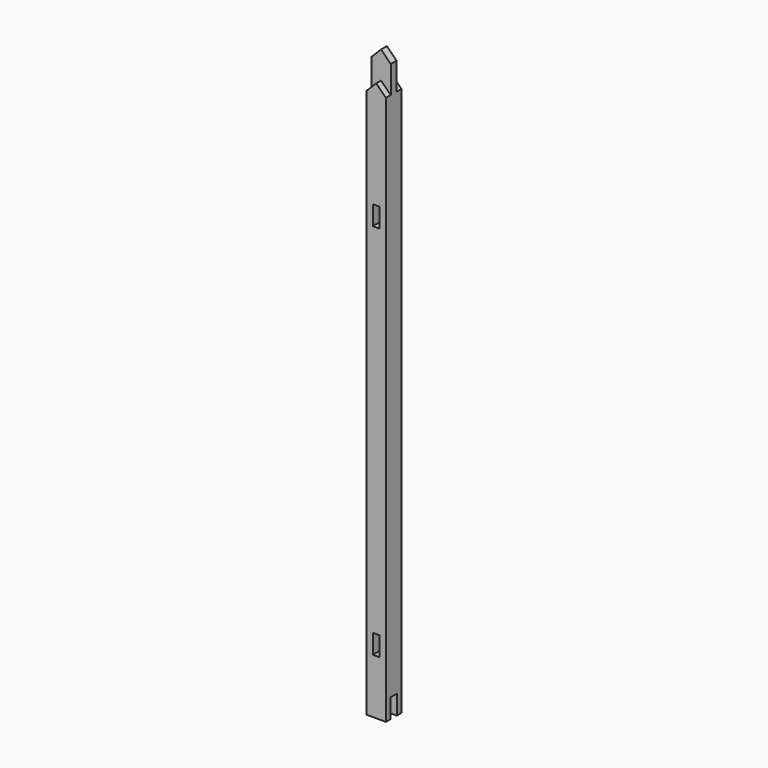
from build123d import *

# Parameters (mm, degrees)
F0_W      = 45
F0_H      = 45
F1_DEPTH  = 650
F3_DEPTH  = 14
F4_W      = 16
F4_H      = 45
F5_DEPTH  = 45.001
F6_W      = 18
F6_H      = 45
F7_DEPTH  = 45.001
F8_W      = 16
F8_H      = 45
F9_DEPTH  = 45.001
F10_W     = 45
F10_H     = 17
F11_DEPTH = 63.6
F13_DEPTH = 31.001


# Not quite as in the source:
# - a pattern or mirror of a feature is missing from the dataset's text; its kind, count and spacing are read off the source's solid


with BuildPart() as f1:
    # F0 (on Top) → F1 (new body, symmetric)
    with BuildSketch(Plane.XY):
        Rectangle(F0_W, F0_H)
    extrude(amount=F1_DEPTH, both=True)

    # F2 (on face) → F3 (cut)
    with BuildSketch(Plane.XZ.offset(22.5)):
        Polygon((22.5, 650), (0, 650), (22.5, 627.5), align=None)
        Polygon((-22.5, 627.5), (0, 650), (-22.5, 650), align=None)
    f3 = extrude(amount=-F3_DEPTH, mode=Mode.SUBTRACT)

    # F3_copies: F3 across plane
    add(f3.mirror(Plane.ZX), mode=Mode.SUBTRACT)

    # F4 (on face) → F5 (cut, through all)
    with BuildSketch(Plane.XZ.offset(22.5)):
        with Locations((0, -500)):
            Rectangle(F4_W, F4_H)
    extrude(amount=-F5_DEPTH, mode=Mode.SUBTRACT)

    # F6 (on face) → F7 (cut, through all)
    with BuildSketch(Plane.YZ.offset(22.5)):
        with Locations((0, -627.5)):
            Rectangle(F6_W, F6_H)
    extrude(amount=-F7_DEPTH, mode=Mode.SUBTRACT)

    # F8 (on face) → F9 (cut, through all)
    with BuildSketch(Plane.XZ.offset(22.5)):
        with Locations((0, 377.5)):
            Rectangle(F8_W, F8_H)
    extrude(amount=-F9_DEPTH, mode=Mode.SUBTRACT)

    # F10 (on face) → F11 (join)
    with BuildSketch(Plane.XY.offset(650)):
        Rectangle(F10_W, F10_H)
    extrude(amount=F11_DEPTH)

    # F12 (on face) → F13 (cut, through all)
    with BuildSketch(Plane.XZ.offset(8.5)):
        Polygon((-22.5, 691.1), (0, 713.6), (-22.5, 713.6), align=None)
        Polygon((22.5, 713.6), (0, 713.6), (22.5, 691.1), align=None)
    extrude(amount=-F13_DEPTH, mode=Mode.SUBTRACT)


solid = f1.part
